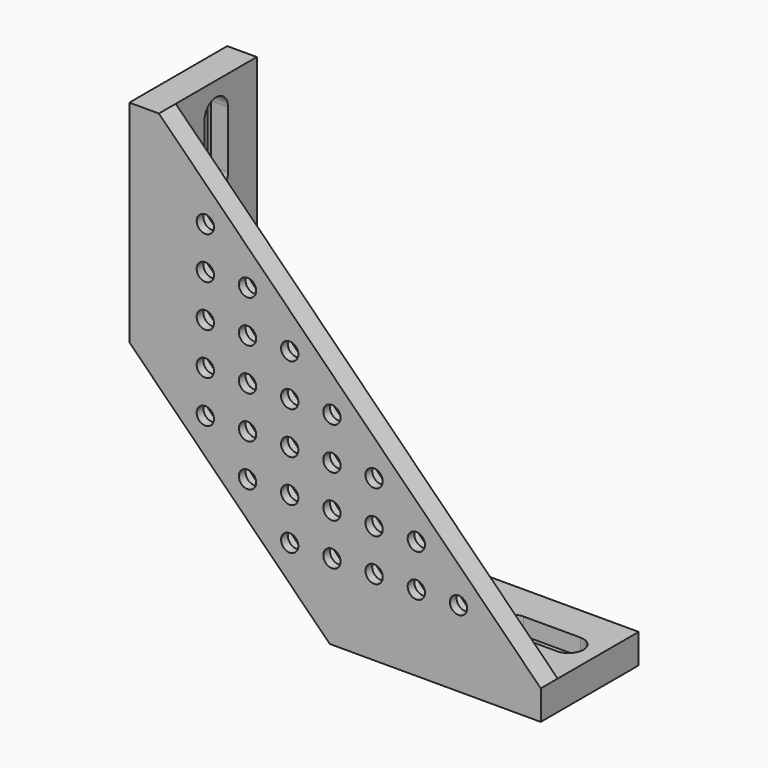
from build123d import *

# Parameters (mm, degrees)
F1_DEPTH  = 7
F2_DEPTH  = 3
F4_ANGLE  = 90
F8_ANGLE  = 180
F12_R     = 2.05
F13_DEPTH = 5
F14_DEPTH = 3


# Not quite as in the source:
# - a feature names something its author has since deleted; it is built from what else it names


with BuildPart() as f1:
    # F0 (on Top) → F1 (new body)
    with BuildSketch(Plane.XY):
        Polygon((29, 12), (-21, 12), (-21, -12), (0, -12), (29, -12), align=None)
        with BuildLine():
            ThreePointArc((-14, -11.5), (-17.5, -8), (-14, -4.5))
            Line((-14, -4.5), (4.5937658288, -4.5))
            Line((4.5937658288, -4.5), (22, -4.5))
            ThreePointArc((22, -4.5), (25.5, -8), (22, -11.5))
            Line((22, -11.5), (5, -11.5))
            Line((5, -11.5), (-14, -11.5))
        make_face(mode=Mode.SUBTRACT)
        with BuildLine():
            Line((-0.5, -3.5), (-14, -3.5))
            ThreePointArc((-14, -3.5), (-17.5, 0), (-14, 3.5))
            Line((-14, 3.5), (-0.5, 3.5))
            Line((-0.5, 3.5), (8.5, 3.5))
            Line((8.5, 3.5), (22, 3.5))
            ThreePointArc((22, 3.5), (25.5, 0), (22, -3.5))
            Line((22, -3.5), (8.5, -3.5))
            Line((8.5, -3.5), (-0.5, -3.5))
        make_face(mode=Mode.SUBTRACT)
        with BuildLine():
            Line((-3, 4.5), (-14, 4.5))
            ThreePointArc((-14, 4.5), (-17.5, 8), (-14, 11.5))
            Line((-14, 11.5), (-3, 11.5))
            Line((-3, 11.5), (22, 11.5))
            ThreePointArc((22, 11.5), (25.5, 8), (22, 4.5))
            Line((22, 4.5), (-3, 4.5))
        make_face(mode=Mode.SUBTRACT)
        with BuildLine():
            Line((4.5937658288, -4.5), (-14, -4.5))
            ThreePointArc((-14, -4.5), (-17.5, -8), (-14, -11.5))
            Line((-14, -11.5), (5, -11.5))
            Line((5, -11.5), (22, -11.5))
            ThreePointArc((22, -11.5), (25.5, -8), (22, -4.5))
            Line((22, -4.5), (4.5937658288, -4.5))
        make_face()
        with BuildLine():
            ThreePointArc((-14, -10.05), (-16.05, -8), (-14, -5.95))
            Line((-14, -5.95), (0, -5.95))
            Line((0, -5.95), (22, -5.95))
            ThreePointArc((22, -5.95), (24.05, -8), (22, -10.05))
            Line((22, -10.05), (0, -10.05))
            Line((0, -10.05), (-14, -10.05))
        make_face(mode=Mode.SUBTRACT)
        with BuildLine():
            ThreePointArc((-14, 11.5), (-17.5, 8), (-14, 4.5))
            Line((-14, 4.5), (-3, 4.5))
            Line((-3, 4.5), (22, 4.5))
            ThreePointArc((22, 4.5), (25.5, 8), (22, 11.5))
            Line((22, 11.5), (-3, 11.5))
            Line((-3, 11.5), (-14, 11.5))
        make_face()
        with BuildLine():
            Line((22, 5.95), (0, 5.95))
            Line((0, 5.95), (-14, 5.95))
            ThreePointArc((-14, 5.95), (-16.05, 8), (-14, 10.05))
            Line((-14, 10.05), (0, 10.05))
            Line((0, 10.05), (22, 10.05))
            ThreePointArc((22, 10.05), (24.05, 8), (22, 5.95))
        make_face(mode=Mode.SUBTRACT)
        with BuildLine():
            Line((0, -5.95), (-14, -5.95))
            ThreePointArc((-14, -5.95), (-16.05, -8), (-14, -10.05))
            Line((-14, -10.05), (0, -10.05))
            Line((0, -10.05), (22, -10.05))
            ThreePointArc((22, -10.05), (24.05, -8), (22, -5.95))
            Line((22, -5.95), (0, -5.95))
        make_face()
        with BuildLine():
            Line((-14, 5.95), (0, 5.95))
            Line((0, 5.95), (22, 5.95))
            ThreePointArc((22, 5.95), (24.05, 8), (22, 10.05))
            Line((22, 10.05), (0, 10.05))
            Line((0, 10.05), (-14, 10.05))
            ThreePointArc((-14, 10.05), (-16.05, 8), (-14, 5.95))
        make_face()
        with BuildLine():
            ThreePointArc((-0.5, 3.5), (3, 0), (-0.5, -3.5))
            Line((-0.5, -3.5), (8.5, -3.5))
            ThreePointArc((8.5, -3.5), (5, 0), (8.5, 3.5))
            Line((8.5, 3.5), (-0.5, 3.5))
        make_face()
    extrude(amount=F1_DEPTH)

    # F0 (on Top) → F2 (join)
    with BuildSketch(Plane.XY):
        with BuildLine():
            ThreePointArc((-14, 3.5), (-17.5, 0), (-14, -3.5))
            Line((-14, -3.5), (-0.5, -3.5))
            ThreePointArc((-0.5, -3.5), (3, 0), (-0.5, 3.5))
            Line((-0.5, 3.5), (-14, 3.5))
        make_face()
        with BuildLine():
            Line((-0.5, -2.45), (-14, -2.45))
            ThreePointArc((-14, -2.45), (-16.45, 0), (-14, 2.45))
            Line((-14, 2.45), (-0.5, 2.45))
            ThreePointArc((-0.5, 2.45), (1.95, 0), (-0.5, -2.45))
        make_face(mode=Mode.SUBTRACT)
        with BuildLine():
            ThreePointArc((8.5, 3.5), (5, 0), (8.5, -3.5))
            Line((8.5, -3.5), (22, -3.5))
            ThreePointArc((22, -3.5), (25.5, 0), (22, 3.5))
            Line((22, 3.5), (8.5, 3.5))
        make_face()
        with BuildLine():
            ThreePointArc((22, 2.45), (24.45, 0), (22, -2.45))
            Line((22, -2.45), (8.5, -2.45))
            ThreePointArc((8.5, -2.45), (6.05, 0), (8.5, 2.45))
            Line((8.5, 2.45), (22, 2.45))
        make_face(mode=Mode.SUBTRACT)
    extrude(amount=F2_DEPTH)


with BuildPart() as f4_1:
    # F4: copy of F1
    add(f1.part.rotate(Axis((-21, 0, 3.5), (0, -1, 0)), F4_ANGLE))


with BuildPart() as f4_1_1:
    # F8: moved
    add(f4_1.part.rotate(Axis((-21, 0, 28.5), (0, 0, 1)), F8_ANGLE))


with BuildPart() as f4_1_2:
    # F9: moved
    add(f4_1_1.part.moved(Location((0, 0, 44))))


with BuildPart() as f4_1_3:
    # F10: moved
    add(f4_1_2.part.moved(Location((-44, 0, 0))))


with BuildPart() as f1_1:
    add(f1.part)

    add(f4_1_3.part)  # F13 merges F4_1
    # F12 (on 3pt) → F13 (join)
    with BuildSketch(Plane.XZ.offset(12)):
        Polygon((-68.5, 47.5), (-21, 0), (29, 0), (29, 7), (-61.5, 97.5), (-68.5, 97.5), align=None)
        Polygon((-34.3563439923, 16.9720831325), (-33.3210678119, 20.8357864376), (-29.4573645067, 21.871062618), (-26.628937382, 19.0426354933), (-27.6642135624, 15.1789321881), (-31.5279168675, 14.1436560077), align=None, mode=Mode.SUBTRACT)
        Polygon((-24.3563439923, 16.9720831325), (-23.3210678119, 20.8357864376), (-19.4573645067, 21.871062618), (-16.628937382, 19.0426354933), (-17.6642135624, 15.1789321881), (-21.5279168675, 14.1436560077), align=None, mode=Mode.SUBTRACT)
        Polygon((-54.3563439923, 36.9720831325), (-53.3210678119, 40.8357864376), (-49.4573645067, 41.871062618), (-46.628937382, 39.0426354933), (-47.6642135624, 35.1789321881), (-51.5279168675, 34.1436560077), align=None, mode=Mode.SUBTRACT)
        Polygon((-54.3563439923, 46.9720831325), (-53.3210678119, 50.8357864376), (-49.4573645067, 51.871062618), (-46.628937382, 49.0426354933), (-47.6642135624, 45.1789321881), (-51.5279168675, 44.1436560077), align=None, mode=Mode.SUBTRACT)
        Polygon((-44.3563439923, 26.9720831325), (-43.3210678119, 30.8357864376), (-39.4573645067, 31.871062618), (-36.628937382, 29.0426354933), (-37.6642135624, 25.1789321881), (-41.5279168675, 24.1436560077), align=None, mode=Mode.SUBTRACT)
        Polygon((-34.3563439923, 26.9720831325), (-33.3210678119, 30.8357864376), (-29.4573645067, 31.871062618), (-26.628937382, 29.0426354933), (-27.6642135624, 25.1789321881), (-31.5279168675, 24.1436560077), align=None, mode=Mode.SUBTRACT)
        Polygon((-24.3563439923, 26.9720831325), (-23.3210678119, 30.8357864376), (-19.4573645067, 31.871062618), (-16.628937382, 29.0426354933), (-17.6642135624, 25.1789321881), (-21.5279168675, 24.1436560077), align=None, mode=Mode.SUBTRACT)
        Polygon((-44.3563439923, 36.9720831325), (-43.3210678119, 40.8357864376), (-39.4573645067, 41.871062618), (-36.628937382, 39.0426354933), (-37.6642135624, 35.1789321881), (-41.5279168675, 34.1436560077), align=None, mode=Mode.SUBTRACT)
        Polygon((-44.3563439923, 46.9720831325), (-43.3210678119, 50.8357864376), (-39.4573645067, 51.871062618), (-36.628937382, 49.0426354933), (-37.6642135624, 45.1789321881), (-41.5279168675, 44.1436560077), align=None, mode=Mode.SUBTRACT)
        Polygon((-34.3563439923, 36.9720831325), (-33.3210678119, 40.8357864376), (-29.4573645067, 41.871062618), (-26.628937382, 39.0426354933), (-27.6642135624, 35.1789321881), (-31.5279168675, 34.1436560077), align=None, mode=Mode.SUBTRACT)
        Polygon((-24.3563439923, 36.9720831325), (-23.3210678119, 40.8357864376), (-19.4573645067, 41.871062618), (-16.628937382, 39.0426354933), (-17.6642135624, 35.1789321881), (-21.5279168675, 34.1436560077), align=None, mode=Mode.SUBTRACT)
        Polygon((-34.3563439923, 46.9720831325), (-33.3210678119, 50.8357864376), (-29.4573645067, 51.871062618), (-26.628937382, 49.0426354933), (-27.6642135624, 45.1789321881), (-31.5279168675, 44.1436560077), align=None, mode=Mode.SUBTRACT)
        Polygon((-24.3563439923, 46.9720831325), (-23.3210678119, 50.8357864376), (-19.4573645067, 51.871062618), (-16.628937382, 49.0426354933), (-17.6642135624, 45.1789321881), (-21.5279168675, 44.1436560077), align=None, mode=Mode.SUBTRACT)
        Polygon((-14.3563439923, 16.9720831325), (-13.3210678119, 20.8357864376), (-9.4573645067, 21.871062618), (-6.628937382, 19.0426354933), (-7.6642135624, 15.1789321881), (-11.5279168675, 14.1436560077), align=None, mode=Mode.SUBTRACT)
        Polygon((-4.3563439923, 16.9720831325), (-3.3210678119, 20.8357864376), (0.5426354933, 21.871062618), (3.371062618, 19.0426354933), (2.3357864376, 15.1789321881), (-1.5279168675, 14.1436560077), align=None, mode=Mode.SUBTRACT)
        Polygon((8.4720831325, 14.1436560077), (5.6436560077, 16.9720831325), (6.6789321881, 20.8357864376), (10.5426354933, 21.871062618), (13.371062618, 19.0426354933), (12.3357864376, 15.1789321881), align=None, mode=Mode.SUBTRACT)
        Polygon((-14.3563439923, 26.9720831325), (-13.3210678119, 30.8357864376), (-9.4573645067, 31.871062618), (-6.628937382, 29.0426354933), (-7.6642135624, 25.1789321881), (-11.5279168675, 24.1436560077), align=None, mode=Mode.SUBTRACT)
        Polygon((-4.3563439923, 26.9720831325), (-3.3210678119, 30.8357864376), (0.5426354933, 31.871062618), (3.371062618, 29.0426354933), (2.3357864376, 25.1789321881), (-1.5279168675, 24.1436560077), align=None, mode=Mode.SUBTRACT)
        Polygon((-14.3563439923, 36.9720831325), (-13.3210678119, 40.8357864376), (-9.4573645067, 41.871062618), (-6.628937382, 39.0426354933), (-7.6642135624, 35.1789321881), (-11.5279168675, 34.1436560077), align=None, mode=Mode.SUBTRACT)
        Polygon((-54.3563439923, 56.9720831325), (-53.3210678119, 60.8357864376), (-49.4573645067, 61.871062618), (-46.628937382, 59.0426354933), (-47.6642135624, 55.1789321881), (-51.5279168675, 54.1436560077), align=None, mode=Mode.SUBTRACT)
        Polygon((-54.3563439923, 66.9720831325), (-53.3210678119, 70.8357864376), (-49.4573645067, 71.871062618), (-46.628937382, 69.0426354933), (-47.6642135624, 65.1789321881), (-51.5279168675, 64.1436560077), align=None, mode=Mode.SUBTRACT)
        Polygon((-44.3563439923, 56.9720831325), (-43.3210678119, 60.8357864376), (-39.4573645067, 61.871062618), (-36.628937382, 59.0426354933), (-37.6642135624, 55.1789321881), (-41.5279168675, 54.1436560077), align=None, mode=Mode.SUBTRACT)
        Polygon((-34.3563439923, 56.9720831325), (-33.3210678119, 60.8357864376), (-29.4573645067, 61.871062618), (-26.628937382, 59.0426354933), (-27.6642135624, 55.1789321881), (-31.5279168675, 54.1436560077), align=None, mode=Mode.SUBTRACT)
        Polygon((-41.5279168675, 64.1436560077), (-44.3563439923, 66.9720831325), (-43.3210678119, 70.8357864376), (-39.4573645067, 71.871062618), (-36.628937382, 69.0426354933), (-37.6642135624, 65.1789321881), align=None, mode=Mode.SUBTRACT)
        Polygon((-51.5279168675, 74.1436560077), (-54.3563439923, 76.9720831325), (-53.3210678119, 80.8357864376), (-49.4573645067, 81.871062618), (-46.628937382, 79.0426354933), (-47.6642135624, 75.1789321881), align=None, mode=Mode.SUBTRACT)
        Polygon((-19.4573645067, 51.871062618), (-23.3210678119, 50.8357864376), (-24.3563439923, 46.9720831325), (-21.5279168675, 44.1436560077), (-17.6642135624, 45.1789321881), (-16.628937382, 49.0426354933), align=None)
        with Locations((-20.4926406871, 48.0073593129)):
            Circle(F12_R, mode=Mode.SUBTRACT)
        Polygon((-29.4573645067, 61.871062618), (-33.3210678119, 60.8357864376), (-34.3563439923, 56.9720831325), (-31.5279168675, 54.1436560077), (-27.6642135624, 55.1789321881), (-26.628937382, 59.0426354933), align=None)
        with Locations((-30.4926406871, 58.0073593129)):
            Circle(F12_R, mode=Mode.SUBTRACT)
        Polygon((-29.4573645067, 51.871062618), (-33.3210678119, 50.8357864376), (-34.3563439923, 46.9720831325), (-31.5279168675, 44.1436560077), (-27.6642135624, 45.1789321881), (-26.628937382, 49.0426354933), align=None)
        with Locations((-30.4926406871, 48.0073593129)):
            Circle(F12_R, mode=Mode.SUBTRACT)
        Polygon((-29.4573645067, 41.871062618), (-33.3210678119, 40.8357864376), (-34.3563439923, 36.9720831325), (-31.5279168675, 34.1436560077), (-27.6642135624, 35.1789321881), (-26.628937382, 39.0426354933), align=None)
        with Locations((-30.4926406871, 38.0073593129)):
            Circle(F12_R, mode=Mode.SUBTRACT)
        Polygon((-19.4573645067, 41.871062618), (-23.3210678119, 40.8357864376), (-24.3563439923, 36.9720831325), (-21.5279168675, 34.1436560077), (-17.6642135624, 35.1789321881), (-16.628937382, 39.0426354933), align=None)
        with Locations((-20.4926406871, 38.0073593129)):
            Circle(F12_R, mode=Mode.SUBTRACT)
        Polygon((-9.4573645067, 41.871062618), (-13.3210678119, 40.8357864376), (-14.3563439923, 36.9720831325), (-11.5279168675, 34.1436560077), (-7.6642135624, 35.1789321881), (-6.628937382, 39.0426354933), align=None)
        with Locations((-10.4926406871, 38.0073593129)):
            Circle(F12_R, mode=Mode.SUBTRACT)
        Polygon((-43.3210678119, 70.8357864376), (-44.3563439923, 66.9720831325), (-41.5279168675, 64.1436560077), (-37.6642135624, 65.1789321881), (-36.628937382, 69.0426354933), (-39.4573645067, 71.871062618), align=None)
        with Locations((-40.4926406871, 68.0073593129)):
            Circle(F12_R, mode=Mode.SUBTRACT)
        Polygon((-39.4573645067, 61.871062618), (-43.3210678119, 60.8357864376), (-44.3563439923, 56.9720831325), (-41.5279168675, 54.1436560077), (-37.6642135624, 55.1789321881), (-36.628937382, 59.0426354933), align=None)
        with Locations((-40.4926406871, 58.0073593129)):
            Circle(F12_R, mode=Mode.SUBTRACT)
        Polygon((-39.4573645067, 51.871062618), (-43.3210678119, 50.8357864376), (-44.3563439923, 46.9720831325), (-41.5279168675, 44.1436560077), (-37.6642135624, 45.1789321881), (-36.628937382, 49.0426354933), align=None)
        with Locations((-40.4926406871, 48.0073593129)):
            Circle(F12_R, mode=Mode.SUBTRACT)
        Polygon((-39.4573645067, 41.871062618), (-43.3210678119, 40.8357864376), (-44.3563439923, 36.9720831325), (-41.5279168675, 34.1436560077), (-37.6642135624, 35.1789321881), (-36.628937382, 39.0426354933), align=None)
        with Locations((-40.4926406871, 38.0073593129)):
            Circle(F12_R, mode=Mode.SUBTRACT)
        Polygon((-39.4573645067, 31.871062618), (-43.3210678119, 30.8357864376), (-44.3563439923, 26.9720831325), (-41.5279168675, 24.1436560077), (-37.6642135624, 25.1789321881), (-36.628937382, 29.0426354933), align=None)
        with Locations((-40.4926406871, 28.0073593129)):
            Circle(F12_R, mode=Mode.SUBTRACT)
        Polygon((-29.4573645067, 31.871062618), (-33.3210678119, 30.8357864376), (-34.3563439923, 26.9720831325), (-31.5279168675, 24.1436560077), (-27.6642135624, 25.1789321881), (-26.628937382, 29.0426354933), align=None)
        with Locations((-30.4926406871, 28.0073593129)):
            Circle(F12_R, mode=Mode.SUBTRACT)
        Polygon((-19.4573645067, 31.871062618), (-23.3210678119, 30.8357864376), (-24.3563439923, 26.9720831325), (-21.5279168675, 24.1436560077), (-17.6642135624, 25.1789321881), (-16.628937382, 29.0426354933), align=None)
        with Locations((-20.4926406871, 28.0073593129)):
            Circle(F12_R, mode=Mode.SUBTRACT)
        Polygon((-9.4573645067, 31.871062618), (-13.3210678119, 30.8357864376), (-14.3563439923, 26.9720831325), (-11.5279168675, 24.1436560077), (-7.6642135624, 25.1789321881), (-6.628937382, 29.0426354933), align=None)
        with Locations((-10.4926406871, 28.0073593129)):
            Circle(F12_R, mode=Mode.SUBTRACT)
        Polygon((0.5426354933, 31.871062618), (-3.3210678119, 30.8357864376), (-4.3563439923, 26.9720831325), (-1.5279168675, 24.1436560077), (2.3357864376, 25.1789321881), (3.371062618, 29.0426354933), align=None)
        with Locations((-0.4926406871, 28.0073593129)):
            Circle(F12_R, mode=Mode.SUBTRACT)
        Polygon((-49.4573645067, 61.871062618), (-53.3210678119, 60.8357864376), (-54.3563439923, 56.9720831325), (-51.5279168675, 54.1436560077), (-47.6642135624, 55.1789321881), (-46.628937382, 59.0426354933), align=None)
        with Locations((-50.4926406871, 58.0073593129)):
            Circle(F12_R, mode=Mode.SUBTRACT)
        Polygon((-49.4573645067, 71.871062618), (-53.3210678119, 70.8357864376), (-54.3563439923, 66.9720831325), (-51.5279168675, 64.1436560077), (-47.6642135624, 65.1789321881), (-46.628937382, 69.0426354933), align=None)
        with Locations((-50.4926406871, 68.0073593129)):
            Circle(F12_R, mode=Mode.SUBTRACT)
        Polygon((-53.3210678119, 80.8357864376), (-54.3563439923, 76.9720831325), (-51.5279168675, 74.1436560077), (-47.6642135624, 75.1789321881), (-46.628937382, 79.0426354933), (-49.4573645067, 81.871062618), align=None)
        with Locations((-50.4926406871, 78.0073593129)):
            Circle(F12_R, mode=Mode.SUBTRACT)
        Polygon((-49.4573645067, 51.871062618), (-53.3210678119, 50.8357864376), (-54.3563439923, 46.9720831325), (-51.5279168675, 44.1436560077), (-47.6642135624, 45.1789321881), (-46.628937382, 49.0426354933), align=None)
        with Locations((-50.4926406871, 48.0073593129)):
            Circle(F12_R, mode=Mode.SUBTRACT)
        Polygon((-49.4573645067, 41.871062618), (-53.3210678119, 40.8357864376), (-54.3563439923, 36.9720831325), (-51.5279168675, 34.1436560077), (-47.6642135624, 35.1789321881), (-46.628937382, 39.0426354933), align=None)
        with Locations((-50.4926406871, 38.0073593129)):
            Circle(F12_R, mode=Mode.SUBTRACT)
        Polygon((-29.4573645067, 21.871062618), (-33.3210678119, 20.8357864376), (-34.3563439923, 16.9720831325), (-31.5279168675, 14.1436560077), (-27.6642135624, 15.1789321881), (-26.628937382, 19.0426354933), align=None)
        with Locations((-30.4926406871, 18.0073593129)):
            Circle(F12_R, mode=Mode.SUBTRACT)
        Polygon((-19.4573645067, 21.871062618), (-23.3210678119, 20.8357864376), (-24.3563439923, 16.9720831325), (-21.5279168675, 14.1436560077), (-17.6642135624, 15.1789321881), (-16.628937382, 19.0426354933), align=None)
        with Locations((-20.4926406871, 18.0073593129)):
            Circle(F12_R, mode=Mode.SUBTRACT)
        Polygon((-9.4573645067, 21.871062618), (-13.3210678119, 20.8357864376), (-14.3563439923, 16.9720831325), (-11.5279168675, 14.1436560077), (-7.6642135624, 15.1789321881), (-6.628937382, 19.0426354933), align=None)
        with Locations((-10.4926406871, 18.0073593129)):
            Circle(F12_R, mode=Mode.SUBTRACT)
        Polygon((0.5426354933, 21.871062618), (-3.3210678119, 20.8357864376), (-4.3563439923, 16.9720831325), (-1.5279168675, 14.1436560077), (2.3357864376, 15.1789321881), (3.371062618, 19.0426354933), align=None)
        with Locations((-0.4926406871, 18.0073593129)):
            Circle(F12_R, mode=Mode.SUBTRACT)
        Polygon((6.6789321881, 20.8357864376), (5.6436560077, 16.9720831325), (8.4720831325, 14.1436560077), (12.3357864376, 15.1789321881), (13.371062618, 19.0426354933), (10.5426354933, 21.871062618), align=None)
        with Locations((9.5073593129, 18.0073593129)):
            Circle(F12_R, mode=Mode.SUBTRACT)
    extrude(amount=F13_DEPTH)

    # F12 (on 3pt) → F14 (cut)
    with BuildSketch(Plane.XZ.offset(12)):
        Polygon((-19.4573645067, 51.871062618), (-23.3210678119, 50.8357864376), (-24.3563439923, 46.9720831325), (-21.5279168675, 44.1436560077), (-17.6642135624, 45.1789321881), (-16.628937382, 49.0426354933), align=None)
        with Locations((-20.4926406871, 48.0073593129)):
            Circle(F12_R, mode=Mode.SUBTRACT)
        Polygon((-9.4573645067, 41.871062618), (-13.3210678119, 40.8357864376), (-14.3563439923, 36.9720831325), (-11.5279168675, 34.1436560077), (-7.6642135624, 35.1789321881), (-6.628937382, 39.0426354933), align=None)
        with Locations((-10.4926406871, 38.0073593129)):
            Circle(F12_R, mode=Mode.SUBTRACT)
        Polygon((-19.4573645067, 41.871062618), (-23.3210678119, 40.8357864376), (-24.3563439923, 36.9720831325), (-21.5279168675, 34.1436560077), (-17.6642135624, 35.1789321881), (-16.628937382, 39.0426354933), align=None)
        with Locations((-20.4926406871, 38.0073593129)):
            Circle(F12_R, mode=Mode.SUBTRACT)
        Polygon((-29.4573645067, 41.871062618), (-33.3210678119, 40.8357864376), (-34.3563439923, 36.9720831325), (-31.5279168675, 34.1436560077), (-27.6642135624, 35.1789321881), (-26.628937382, 39.0426354933), align=None)
        with Locations((-30.4926406871, 38.0073593129)):
            Circle(F12_R, mode=Mode.SUBTRACT)
        Polygon((-29.4573645067, 51.871062618), (-33.3210678119, 50.8357864376), (-34.3563439923, 46.9720831325), (-31.5279168675, 44.1436560077), (-27.6642135624, 45.1789321881), (-26.628937382, 49.0426354933), align=None)
        with Locations((-30.4926406871, 48.0073593129)):
            Circle(F12_R, mode=Mode.SUBTRACT)
        Polygon((-29.4573645067, 61.871062618), (-33.3210678119, 60.8357864376), (-34.3563439923, 56.9720831325), (-31.5279168675, 54.1436560077), (-27.6642135624, 55.1789321881), (-26.628937382, 59.0426354933), align=None)
        with Locations((-30.4926406871, 58.0073593129)):
            Circle(F12_R, mode=Mode.SUBTRACT)
        Polygon((0.5426354933, 31.871062618), (-3.3210678119, 30.8357864376), (-4.3563439923, 26.9720831325), (-1.5279168675, 24.1436560077), (2.3357864376, 25.1789321881), (3.371062618, 29.0426354933), align=None)
        with Locations((-0.4926406871, 28.0073593129)):
            Circle(F12_R, mode=Mode.SUBTRACT)
        Polygon((-9.4573645067, 31.871062618), (-13.3210678119, 30.8357864376), (-14.3563439923, 26.9720831325), (-11.5279168675, 24.1436560077), (-7.6642135624, 25.1789321881), (-6.628937382, 29.0426354933), align=None)
        with Locations((-10.4926406871, 28.0073593129)):
            Circle(F12_R, mode=Mode.SUBTRACT)
        Polygon((-19.4573645067, 31.871062618), (-23.3210678119, 30.8357864376), (-24.3563439923, 26.9720831325), (-21.5279168675, 24.1436560077), (-17.6642135624, 25.1789321881), (-16.628937382, 29.0426354933), align=None)
        with Locations((-20.4926406871, 28.0073593129)):
            Circle(F12_R, mode=Mode.SUBTRACT)
        Polygon((-29.4573645067, 31.871062618), (-33.3210678119, 30.8357864376), (-34.3563439923, 26.9720831325), (-31.5279168675, 24.1436560077), (-27.6642135624, 25.1789321881), (-26.628937382, 29.0426354933), align=None)
        with Locations((-30.4926406871, 28.0073593129)):
            Circle(F12_R, mode=Mode.SUBTRACT)
        Polygon((-39.4573645067, 31.871062618), (-43.3210678119, 30.8357864376), (-44.3563439923, 26.9720831325), (-41.5279168675, 24.1436560077), (-37.6642135624, 25.1789321881), (-36.628937382, 29.0426354933), align=None)
        with Locations((-40.4926406871, 28.0073593129)):
            Circle(F12_R, mode=Mode.SUBTRACT)
        Polygon((-39.4573645067, 41.871062618), (-43.3210678119, 40.8357864376), (-44.3563439923, 36.9720831325), (-41.5279168675, 34.1436560077), (-37.6642135624, 35.1789321881), (-36.628937382, 39.0426354933), align=None)
        with Locations((-40.4926406871, 38.0073593129)):
            Circle(F12_R, mode=Mode.SUBTRACT)
        Polygon((-39.4573645067, 51.871062618), (-43.3210678119, 50.8357864376), (-44.3563439923, 46.9720831325), (-41.5279168675, 44.1436560077), (-37.6642135624, 45.1789321881), (-36.628937382, 49.0426354933), align=None)
        with Locations((-40.4926406871, 48.0073593129)):
            Circle(F12_R, mode=Mode.SUBTRACT)
        Polygon((-39.4573645067, 61.871062618), (-43.3210678119, 60.8357864376), (-44.3563439923, 56.9720831325), (-41.5279168675, 54.1436560077), (-37.6642135624, 55.1789321881), (-36.628937382, 59.0426354933), align=None)
        with Locations((-40.4926406871, 58.0073593129)):
            Circle(F12_R, mode=Mode.SUBTRACT)
        Polygon((-43.3210678119, 70.8357864376), (-44.3563439923, 66.9720831325), (-41.5279168675, 64.1436560077), (-37.6642135624, 65.1789321881), (-36.628937382, 69.0426354933), (-39.4573645067, 71.871062618), align=None)
        with Locations((-40.4926406871, 68.0073593129)):
            Circle(F12_R, mode=Mode.SUBTRACT)
        Polygon((-53.3210678119, 80.8357864376), (-54.3563439923, 76.9720831325), (-51.5279168675, 74.1436560077), (-47.6642135624, 75.1789321881), (-46.628937382, 79.0426354933), (-49.4573645067, 81.871062618), align=None)
        with Locations((-50.4926406871, 78.0073593129)):
            Circle(F12_R, mode=Mode.SUBTRACT)
        Polygon((-49.4573645067, 71.871062618), (-53.3210678119, 70.8357864376), (-54.3563439923, 66.9720831325), (-51.5279168675, 64.1436560077), (-47.6642135624, 65.1789321881), (-46.628937382, 69.0426354933), align=None)
        with Locations((-50.4926406871, 68.0073593129)):
            Circle(F12_R, mode=Mode.SUBTRACT)
        Polygon((-49.4573645067, 61.871062618), (-53.3210678119, 60.8357864376), (-54.3563439923, 56.9720831325), (-51.5279168675, 54.1436560077), (-47.6642135624, 55.1789321881), (-46.628937382, 59.0426354933), align=None)
        with Locations((-50.4926406871, 58.0073593129)):
            Circle(F12_R, mode=Mode.SUBTRACT)
        Polygon((-49.4573645067, 51.871062618), (-53.3210678119, 50.8357864376), (-54.3563439923, 46.9720831325), (-51.5279168675, 44.1436560077), (-47.6642135624, 45.1789321881), (-46.628937382, 49.0426354933), align=None)
        with Locations((-50.4926406871, 48.0073593129)):
            Circle(F12_R, mode=Mode.SUBTRACT)
        Polygon((-49.4573645067, 41.871062618), (-53.3210678119, 40.8357864376), (-54.3563439923, 36.9720831325), (-51.5279168675, 34.1436560077), (-47.6642135624, 35.1789321881), (-46.628937382, 39.0426354933), align=None)
        with Locations((-50.4926406871, 38.0073593129)):
            Circle(F12_R, mode=Mode.SUBTRACT)
        Polygon((-29.4573645067, 21.871062618), (-33.3210678119, 20.8357864376), (-34.3563439923, 16.9720831325), (-31.5279168675, 14.1436560077), (-27.6642135624, 15.1789321881), (-26.628937382, 19.0426354933), align=None)
        with Locations((-30.4926406871, 18.0073593129)):
            Circle(F12_R, mode=Mode.SUBTRACT)
        Polygon((-19.4573645067, 21.871062618), (-23.3210678119, 20.8357864376), (-24.3563439923, 16.9720831325), (-21.5279168675, 14.1436560077), (-17.6642135624, 15.1789321881), (-16.628937382, 19.0426354933), align=None)
        with Locations((-20.4926406871, 18.0073593129)):
            Circle(F12_R, mode=Mode.SUBTRACT)
        Polygon((-9.4573645067, 21.871062618), (-13.3210678119, 20.8357864376), (-14.3563439923, 16.9720831325), (-11.5279168675, 14.1436560077), (-7.6642135624, 15.1789321881), (-6.628937382, 19.0426354933), align=None)
        with Locations((-10.4926406871, 18.0073593129)):
            Circle(F12_R, mode=Mode.SUBTRACT)
        Polygon((0.5426354933, 21.871062618), (-3.3210678119, 20.8357864376), (-4.3563439923, 16.9720831325), (-1.5279168675, 14.1436560077), (2.3357864376, 15.1789321881), (3.371062618, 19.0426354933), align=None)
        with Locations((-0.4926406871, 18.0073593129)):
            Circle(F12_R, mode=Mode.SUBTRACT)
        Polygon((6.6789321881, 20.8357864376), (5.6436560077, 16.9720831325), (8.4720831325, 14.1436560077), (12.3357864376, 15.1789321881), (13.371062618, 19.0426354933), (10.5426354933, 21.871062618), align=None)
        with Locations((9.5073593129, 18.0073593129)):
            Circle(F12_R, mode=Mode.SUBTRACT)
    extrude(amount=F14_DEPTH, mode=Mode.SUBTRACT)


solid = f1_1.part
